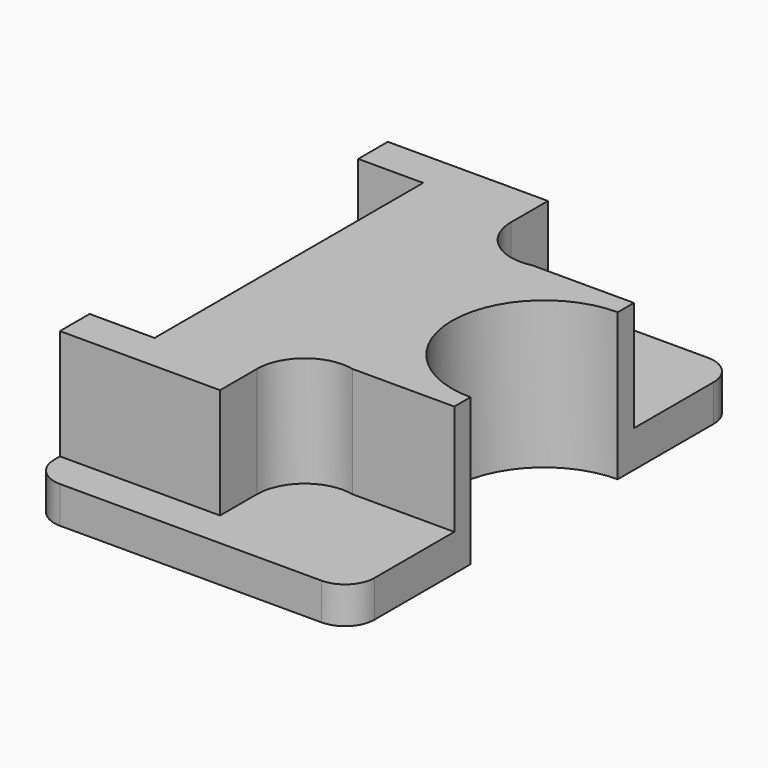
from build123d import *

# Parameters (mm, degrees)
F0_W     = 55.290274322
F0_H     = 83.3742246032
F1_DEPTH = 25.4
F2_R     = 15.8926372782
F3_DEPTH = 25.401
F4_W     = 11.2183341355
F4_H     = 57.9742246032
F5_DEPTH = 19.05
F7_DEPTH = 19.05
F8_R     = 5.08


# Not quite as in the source:
# - a pattern or mirror of a feature is missing from the dataset's text; its kind, count and spacing are read off the source's solid


with BuildPart() as f1:
    # F0 (on Top) → F1 (new body)
    with BuildSketch(Plane.XY):
        Rectangle(F0_W, F0_H)
    extrude(amount=F1_DEPTH)

    # F2 (on face) → F3 (cut, through all)
    with BuildSketch(Plane.XY.offset(25.4)):
        with Locations((27.645137161, 0)):
            Circle(F2_R)
    extrude(amount=-F3_DEPTH, mode=Mode.SUBTRACT)

    # F4 (on face) → F5 (cut)
    with BuildSketch(Plane.XY.offset(25.4)):
        with Locations((-22.0359700932, 0)):
            Rectangle(F4_W, F4_H)
    extrude(amount=-F5_DEPTH, mode=Mode.SUBTRACT)

    # F6 (on face) → F7 (cut)
    with BuildSketch(Plane.XY.offset(25.4)):
        with BuildLine():
            Line((27.645137161, -41.6871123016), (27.645137161, -19.3835441023))
            Line((27.645137161, -19.3835441023), (10.0954379886, -19.3835441023))
            ThreePointArc((10.0954379886, -19.3835441023), (3.1118668584, -20.9577512479), (0, -27.4048186839))
            Line((0, -27.4048186839), (0, -35.3843905032))
            Line((0, -35.3843905032), (-27.645137161, -35.3843905032))
            Line((-27.645137161, -35.3843905032), (-27.645137161, -41.6871123016))
            Line((-27.645137161, -41.6871123016), (27.645137161, -41.6871123016))
        make_face()
    f7 = extrude(amount=-F7_DEPTH, mode=Mode.SUBTRACT)

    # F7_copies: F7 across plane
    add(f7.mirror(Plane.ZX), mode=Mode.SUBTRACT)

    # F8
    f8_edges = [f1.edges().sort_by_distance(p)[0] for p in [
        (27.645137, -41.687112, 3.175),
        (27.645137, 41.687112, 3.175),
        (-27.645137, 41.687112, 3.175),
        (-27.645137, -41.687112, 3.175),
    ]]
    fillet(f8_edges, radius=F8_R)


solid = f1.part
